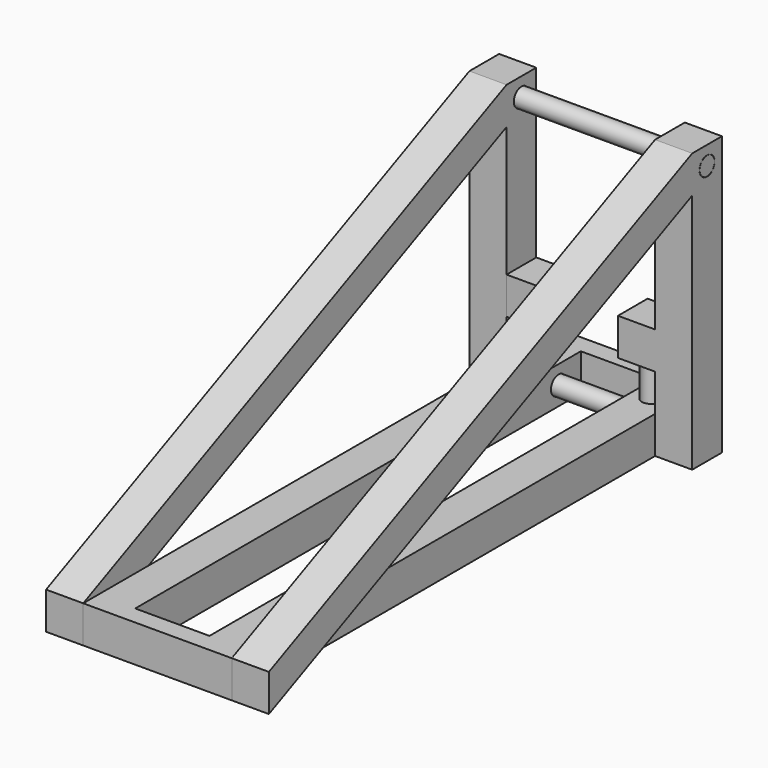
from build123d import *

# Parameters (mm, degrees)
F0_W           = 50.8
F0_H           = 12.7
F1_DEPTH       = 203.2
F2_W           = 25.4
F2_H           = 190.5
F3_DEPTH       = 12.701
F4_R           = 3.2385
F5_DEPTH       = 50.801
F6_R           = 3.175
F7_DEPTH       = 50.8
F9_DEPTH       = 12.7
F11_DEPTH      = 12.7
F12_R          = 3.2385
F13_DEPTH      = 76.201
F14_R          = 3.2385
F15_DEPTH      = 76.201
F16_R          = 3.175
F17_DEPTH      = 76.2
F18_R          = 3.2385
F19_DEPTH      = 3.175
F20_R          = 3.175
F21_DEPTH      = 15.875
F21_DEPTH_BACK = 3.175
F22_W          = 12.7
F22_H          = 12.7
F23_DEPTH      = 12.7
F24_R          = 3.2385
F25_DEPTH      = 3.175
F26_W          = 12.7
F26_H          = 12.7
F27_DEPTH      = 12.7
F28_R          = 3.2385
F29_DEPTH      = 3.175


with BuildPart() as f1:
    # F0 (on Front) → F1 (new body)
    with BuildSketch(Plane.XZ):
        with Locations((25.4, 6.35)):
            Rectangle(F0_W, F0_H)
    extrude(amount=F1_DEPTH)

    # F2 (on face) → F3 (cut, through all)
    with BuildSketch(Plane.XY.offset(12.7)):
        with Locations((25.4, -101.6)):
            Rectangle(F2_W, F2_H)
    extrude(amount=-F3_DEPTH, mode=Mode.SUBTRACT)

    # F4 (on face) → F5 (cut, through all)
    with BuildSketch(Plane.YZ.offset(50.8)):
        with Locations((-15.875, 6.35)):
            Circle(F4_R)
    extrude(amount=-F5_DEPTH, mode=Mode.SUBTRACT)

    # F14 (on face) → F15 (cut, through all)
    with BuildSketch(Plane(origin=(-12.7, 0, 0), x_dir=(0, -1, 0), z_dir=(-1, 0, 0))):
        with Locations((15.875, 88.9)):
            Circle(F14_R)
    extrude(amount=-F15_DEPTH, mode=Mode.SUBTRACT)

    # F18 (on face) → F19 (cut)
    with BuildSketch(Plane.XY.offset(12.7)):
        with Locations((6.35, -15.875)):
            Circle(F18_R)
        with Locations((44.45, -15.875)):
            Circle(F18_R)
    extrude(amount=-F19_DEPTH, mode=Mode.SUBTRACT)


with BuildPart() as f7:
    # F6 (on face) → F7 (new body)
    with BuildSketch(Plane.YZ.offset(50.8)):
        with Locations((-15.875, 6.35)):
            Circle(F6_R)
    extrude(amount=-F7_DEPTH)


with BuildPart() as f9:
    # F8 (on face) → F9 (new body)
    with BuildSketch(Plane.YZ.offset(50.8)):
        Polygon((-22.225, 0), (-9.525, 0), (-9.525, 95.25), (-22.225, 95.25), (-22.225, 82.55), align=None)
        Polygon((-203.2, 0), (-22.225, 82.55), (-22.225, 95.25), (-203.2, 12.7), align=None)
    extrude(amount=F9_DEPTH)


with BuildPart() as f11:
    # F10 (on face) → F11 (new body)
    with BuildSketch(Plane(origin=(0, 0, 0), x_dir=(0, -1, 0), z_dir=(-1, 0, 0))):
        Polygon((9.525, 95.25), (9.525, 0), (22.225, 0), (22.225, 82.55), (22.225, 95.25), align=None)
        Polygon((22.225, 95.25), (22.225, 82.55), (203.2, 0), (203.2, 12.7), align=None)
    extrude(amount=F11_DEPTH)


with BuildPart() as f13_tool:
    # F12 (on face) → F13 (new body, through all)
    with BuildSketch(Plane.YZ.offset(63.5)):
        with Locations((-15.875, 88.9)):
            Circle(F12_R)
    extrude(amount=-F13_DEPTH)


with BuildPart() as f9_1:
    add(f9.part)

    # F13: cut by f13_tool
    add(f13_tool.part, mode=Mode.SUBTRACT)

    # F26 (on face) → F27 (join)
    with BuildSketch(Plane(origin=(50.8, 0, 0), x_dir=(0, -1, 0), z_dir=(-1, 0, 0))):
        with Locations((15.875, 31.75)):
            Rectangle(F26_W, F26_H)
    extrude(amount=F27_DEPTH)

    # F28 (on face) → F29 (cut)
    with BuildSketch(Plane(origin=(0, 0, 25.4), x_dir=(1, 0, 0), z_dir=(0, 0, -1))):
        with Locations((44.45, 15.875)):
            Circle(F28_R)
    extrude(amount=-F29_DEPTH, mode=Mode.SUBTRACT)


with BuildPart() as f11_1:
    add(f11.part)

    # F13: cut by f13_tool
    add(f13_tool.part, mode=Mode.SUBTRACT)


with BuildPart() as f17:
    # F16 (on face) → F17 (new body)
    with BuildSketch(Plane(origin=(-12.7, 0, 0), x_dir=(0, -1, 0), z_dir=(-1, 0, 0))):
        with Locations((15.875, 88.9)):
            Circle(F16_R)
    extrude(amount=-F17_DEPTH)


with BuildPart() as f21:
    # F20 (on face) → F21 (new body, two sides)
    with BuildSketch(Plane.XY.offset(12.7)) as f21_sk:
        with Locations((6.35, -15.875)):
            Circle(F20_R)
    extrude(amount=F21_DEPTH)
    extrude(f21_sk.sketch, amount=-F21_DEPTH_BACK)


with BuildPart() as f21b:
    # F20 (on face) → F21, piece 2 (new body, two sides)
    with BuildSketch(Plane.XY.offset(12.7)) as f21_2_sk:
        with Locations((44.45, -15.875)):
            Circle(F20_R)
    extrude(amount=F21_DEPTH)
    extrude(f21_2_sk.sketch, amount=-F21_DEPTH_BACK)


with BuildPart() as f23:
    # F22 (on face) → F23 (new body)
    with BuildSketch(Plane.YZ):
        with Locations((-15.875, 31.75)):
            Rectangle(F22_W, F22_H)
    extrude(amount=F23_DEPTH)

    # F24 (on face) → F25 (cut)
    with BuildSketch(Plane(origin=(0, 0, 25.4), x_dir=(1, 0, 0), z_dir=(0, 0, -1))):
        with Locations((6.35, 15.875)):
            Circle(F24_R)
    extrude(amount=-F25_DEPTH, mode=Mode.SUBTRACT)


solid = Compound([f1.part, f7.part, f9_1.part, f11_1.part, f17.part, f21.part, f21b.part, f23.part])
